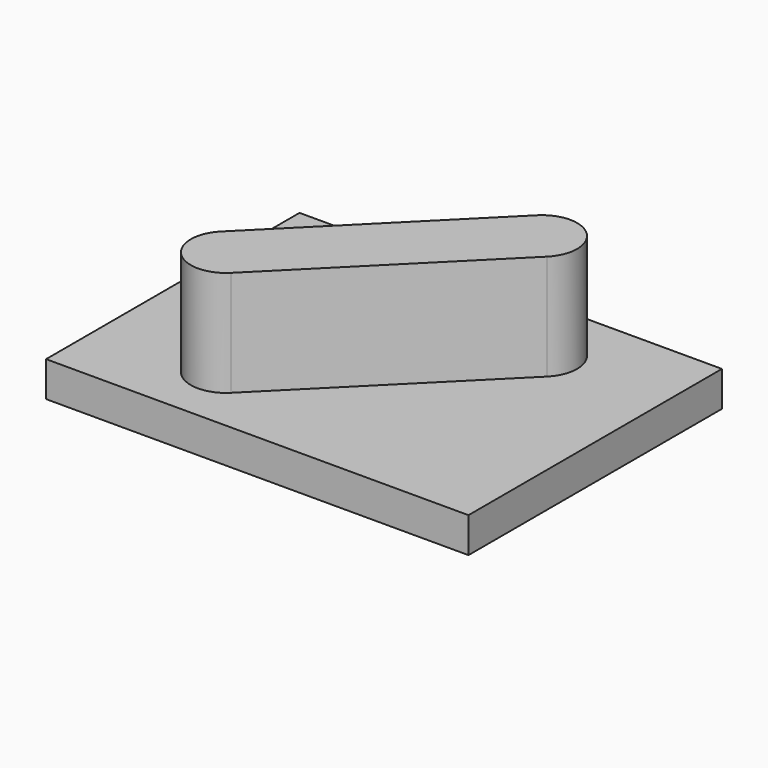
from build123d import *

# Parameters (mm, degrees)
F0_W     = 152.4
F0_H     = 114.3
F1_DEPTH = 6.35
F3_DEPTH = 38.1


with BuildPart() as f1:
    # F0 (on Top) → F1 (new body, symmetric)
    with BuildSketch(Plane.XY):
        with Locations((-76.2, 57.15)):
            Rectangle(F0_W, F0_H)
    extrude(amount=F1_DEPTH, both=True)

    # F2 (on face) → F3 (join)
    with BuildSketch(Plane.XY.offset(6.35)):
        Polygon((-53.5205122421, 97.79), (-116.84, 34.4705122421), (-107.8597438789, 25.4902561211), (-98.8794877579, 16.51), (-35.56, 79.8294877579), (-44.5402561211, 88.8097438789), align=None)
        with BuildLine():
            Line((-107.8597438789, 25.4902561211), (-116.84, 34.4705122421))
            ThreePointArc((-116.84, 34.4705122421), (-116.84, 16.51), (-98.8794877579, 16.51))
            Line((-98.8794877579, 16.51), (-107.8597438789, 25.4902561211))
        make_face()
        with BuildLine():
            ThreePointArc((-35.56, 79.8294877579), (-35.56, 97.79), (-53.5205122421, 97.79))
            Line((-53.5205122421, 97.79), (-44.5402561211, 88.8097438789))
            Line((-44.5402561211, 88.8097438789), (-35.56, 79.8294877579))
        make_face()
    extrude(amount=F3_DEPTH)


solid = f1.part
